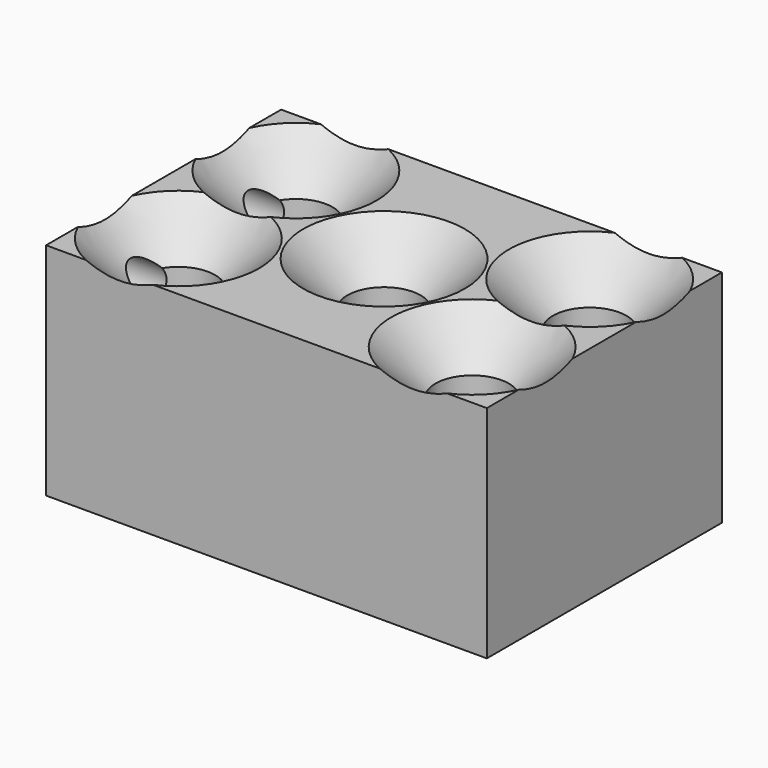
from build123d import *

# Parameters (mm, degrees)
F0_R     = 2.5
F1_DEPTH = 15
F3_R     = 1.5
F4_DEPTH = 5


# Not quite as in the source:
# - a fillet or chamfer that OpenCascade refuses, or shapes differently, is made with other operations: its cross-section is extruded or revolved along the edge and cut away or added


with BuildPart() as f1:
    # F0 (on Top) → F1 (new body)
    with BuildSketch(Plane.XY):
        Polygon((-5, 10), (-15, 10), (-15, 5), (-15, -10), (15, -10), (15, 10), align=None)
        with Locations((-10, -5)):
            Circle(F0_R, mode=Mode.SUBTRACT)
        with Locations((10, -5)):
            Circle(F0_R, mode=Mode.SUBTRACT)
        with BuildLine():
            ThreePointArc((-7.5, 5), (-10, 2.5), (-12.5, 5))
            ThreePointArc((-12.5, 5), (-10, 7.5), (-7.5, 5))
        make_face(mode=Mode.SUBTRACT)
        Circle(F0_R, mode=Mode.SUBTRACT)
        with Locations((10, 5)):
            Circle(F0_R, mode=Mode.SUBTRACT)
    extrude(amount=F1_DEPTH)

    # F2: chamfer of 3 on 5 edges, made by hand

    # F2_s1 → F2_t2 (revolve, cut)
    with BuildSketch(Plane.XZ.offset(-5)):
        Polygon((-4.5, 15), (-7.5, 12), (-7.5, 15), align=None)
    revolve(axis=Axis((-10, 5, 15), (0, 0, 1)), mode=Mode.SUBTRACT)

    # F2_s3 → F2_t4 (revolve, cut)
    with BuildSketch(Plane.XZ):
        Polygon((5.5, 15), (2.5, 12), (2.5, 15), align=None)
    revolve(axis=Axis((0, 0, 15), (0, 0, 1)), mode=Mode.SUBTRACT)

    # F2_s5 → F2_t6 (revolve, cut)
    with BuildSketch(Plane.XZ.offset(5)):
        Polygon((-4.5, 15), (-7.5, 12), (-7.5, 15), align=None)
    revolve(axis=Axis((-10, -5, 15), (0, 0, 1)), mode=Mode.SUBTRACT)

    # F2_s7 → F2_t8 (revolve, cut)
    with BuildSketch(Plane.XZ.offset(-5)):
        Polygon((15.5, 15), (12.5, 12), (12.5, 15), align=None)
    revolve(axis=Axis((10, 5, 15), (0, 0, 1)), mode=Mode.SUBTRACT)

    # F2_s9 → F2_t10 (revolve, cut)
    with BuildSketch(Plane.XZ.offset(5)):
        Polygon((15.5, 15), (12.5, 12), (12.5, 15), align=None)
    revolve(axis=Axis((10, -5, 15), (0, 0, 1)), mode=Mode.SUBTRACT)

    # F3 (on face) → F4 (cut)
    with BuildSketch(Plane(origin=(-15, 0, 0), x_dir=(0, -1, 0), z_dir=(-1, 0, 0))):
        with Locations((0, 7.5)):
            Circle(F3_R)
        with Locations((-5, 11.2557266839)):
            Circle(F3_R)
        with Locations((-5, 3.7442733161)):
            Circle(F3_R)
        with Locations((5, 11.2557266839)):
            Circle(F3_R)
        with Locations((5, 3.7442733161)):
            Circle(F3_R)
    extrude(amount=-F4_DEPTH, mode=Mode.SUBTRACT)


solid = f1.part
